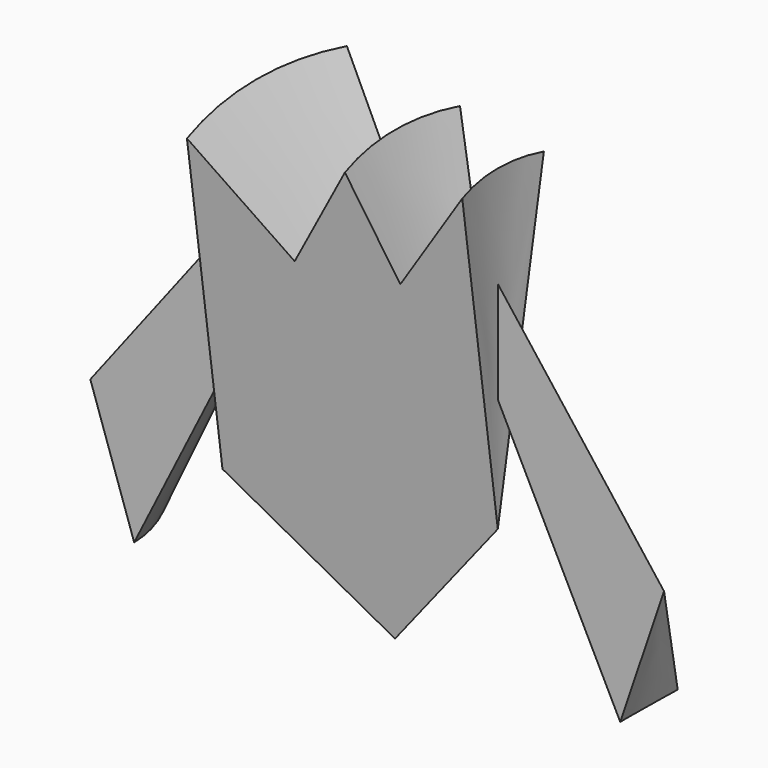
from build123d import *

# Parameters (mm, degrees)
F1_ANGLE_BACK = 15
F1_ANGLE      = 30
F2_ANGLE      = 30
F3_ANGLE      = 30


with BuildPart() as f1:
    # F0 (on Front) → F1 (revolve)
    with BuildSketch(Plane.XZ, mode=Mode.PRIVATE) as f1_sk:
        Polygon((-25.7571255401, 24.1777971488), (0, 0), (19.1233232134, 24.1777971488), (19.1233232134, 45.4059700859), (19.1233232134, 64.3459617069), (19.1233232134, 83.2859533279), (7.2450009175, 65.0988072157), (0, 83.3688080311), (-9.9750002846, 65.0988072157), (-25.7571255401, 83.2859533279), (-25.7571255401, 64.3459617069), (-25.7571255401, 45.4059700859), align=None)
    revolve(f1_sk.sketch.rotate(Axis((9.5616616067, 0, 12.0888985744), (0.6203552442, 0, 0.7843209617)), -F1_ANGLE_BACK), axis=Axis((9.5616616067, 0, 12.0888985744), (0.6203552442, 0, 0.7843209617)), revolution_arc=F1_ANGLE)


with BuildPart() as f2:
    # F0 (on Front) → F2 (revolve)
    with BuildSketch(Plane.XZ):
        Polygon((19.1233232134, 64.3459617069), (19.1233232134, 45.4059700859), (41.9035313019, 0), (50.0620402672, 24.0540793102), align=None)
    revolve(axis=Axis((34.5926817403, 0, 44.2000205086), (0.6090298633, 0, -0.7931472913)), revolution_arc=F2_ANGLE)


with BuildPart() as f3:
    # F0 (on Front) → F3 (revolve)
    with BuildSketch(Plane.XZ):
        Polygon((-48.5373336286, 0), (-25.7571255401, 45.4059700859), (-25.7571255401, 64.3459617069), (-56.6958425939, 24.0540793102), align=None)
    revolve(axis=Axis((-41.226484067, 0, 44.2000205086), (0.6090298633, 0, 0.7931472913)), revolution_arc=F3_ANGLE)


solid = Compound([f1.part, f2.part, f3.part])
